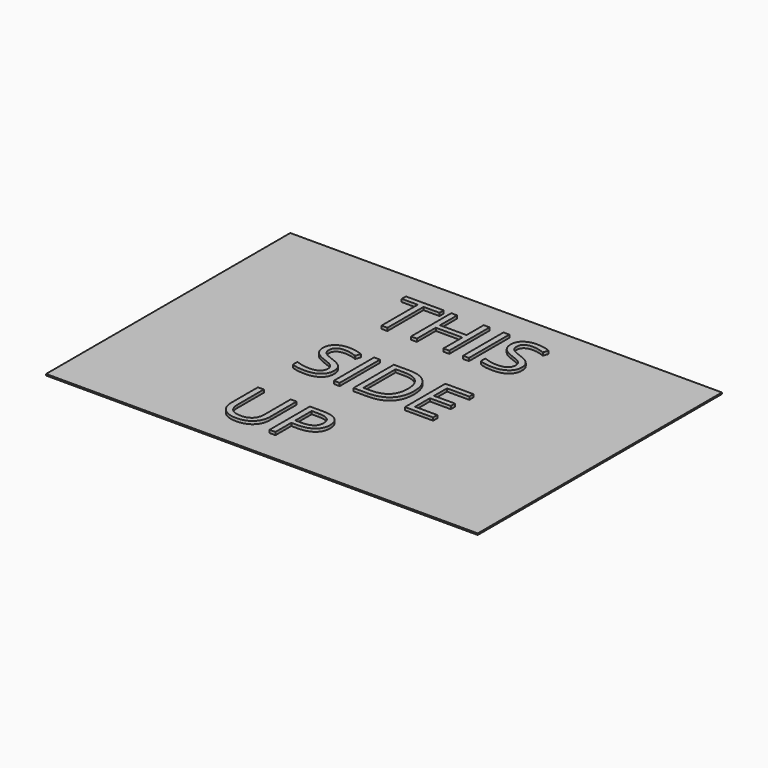
from build123d import *

# Parameters (mm, degrees)
F0_W         = 297
F0_H         = 210
F1_DEPTH     = 1
F2_TEXT_SIZE = 48.6111111111
F3_DEPTH     = 2


# Not quite as in the source:
# - Text() gives the source's letters only with a copy of the font that has no kerning and outlines rounded to 1/6400 em; it was checked with that copy


with BuildPart() as f1:
    # F0 (on Top) → F1 (new body)
    with BuildSketch(Plane.XY):
        with Locations((-103.4256041646, 58.6126293242)):
            Rectangle(F0_W, F0_H)
    extrude(amount=F1_DEPTH)

    # F2 (on face) → F3 (join)
    with BuildSketch(Plane.XY.offset(1)):
        with Locations((-155.3331562479, 107.09897118)):
            Text('THIS', F2_TEXT_SIZE, font='Open Sans', text_align=(TextAlign.LEFT, TextAlign.BOTTOM))
        with Locations((-155.3331562479, 40.9878600689)):
            Text('SIDE', F2_TEXT_SIZE, font='Open Sans', text_align=(TextAlign.LEFT, TextAlign.BOTTOM))
        with Locations((-155.3331562479, -25.1232510423)):
            Text('UP', F2_TEXT_SIZE, font='Open Sans', text_align=(TextAlign.LEFT, TextAlign.BOTTOM))
    extrude(amount=F3_DEPTH)


solid = f1.part
